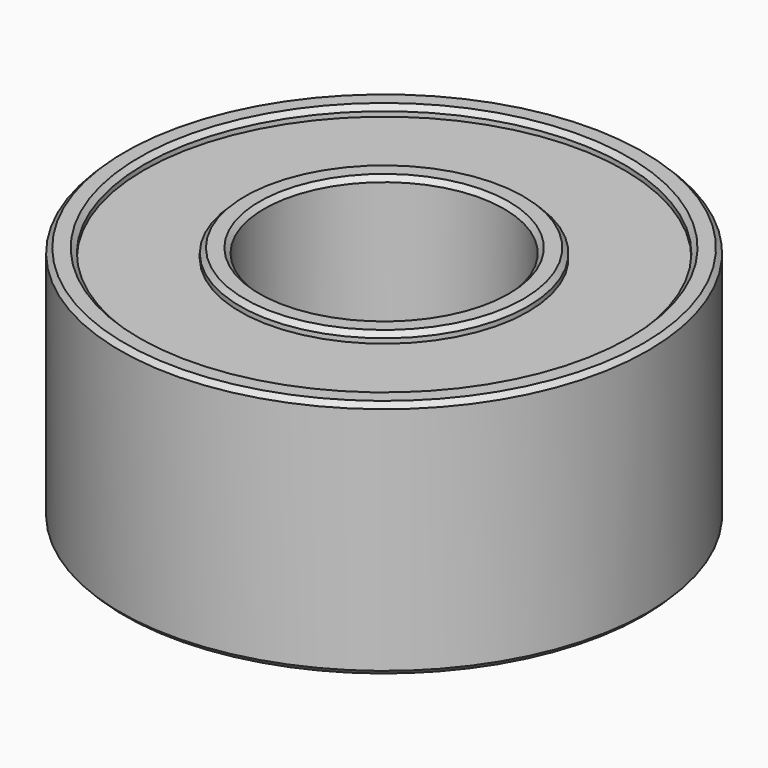
from build123d import *

# Parameters (mm, degrees)
F0_R      = 3
F0_R_2    = 2.5
F1_DEPTH  = 5
F0_R_3    = 5.5
F0_R_4    = 5
F2_START  = 0.2
F2_DEPTH  = 4.6
F3_SIZE   = 0.1
F3_2_SIZE = 0.1


with BuildPart() as f1:
    # F0 (on Top) → F1 (new body)
    with BuildSketch(Plane.XY):
        Circle(F0_R)
        Circle(F0_R_2, mode=Mode.SUBTRACT)
    extrude(amount=F1_DEPTH)

    # F3
    f3_edges = [f1.edges().sort_by_distance(p)[0] for p in [
        (-3, 0, 0),
        (-2.5, 0, 0),
        (-3, 0, 5),
        (-2.5, 0, 5),
    ]]
    chamfer(f3_edges, length=F3_SIZE)


with BuildPart() as f1b:
    # F0 (on Top) → F1, piece 2 (new body)
    with BuildSketch(Plane.XY):
        Circle(F0_R_3)
        Circle(F0_R_4, mode=Mode.SUBTRACT)
    extrude(amount=F1_DEPTH)

    # F3#2
    f3_2_edges = [f1b.edges().sort_by_distance(p)[0] for p in [
        (-5.5, 0, 5),
        (-5, 0, 5),
        (-5.5, 0, 0),
        (-5, 0, 0),
    ]]
    chamfer(f3_2_edges, length=F3_2_SIZE)


with BuildPart() as f2:
    # F0 (on Top) → F2 (new body)
    with BuildSketch(Plane.XY.offset(F2_START)):
        Circle(F0_R_4)
        Circle(F0_R, mode=Mode.SUBTRACT)
    extrude(amount=F2_DEPTH)


solid = Compound([f1.part, f1b.part, f2.part])
